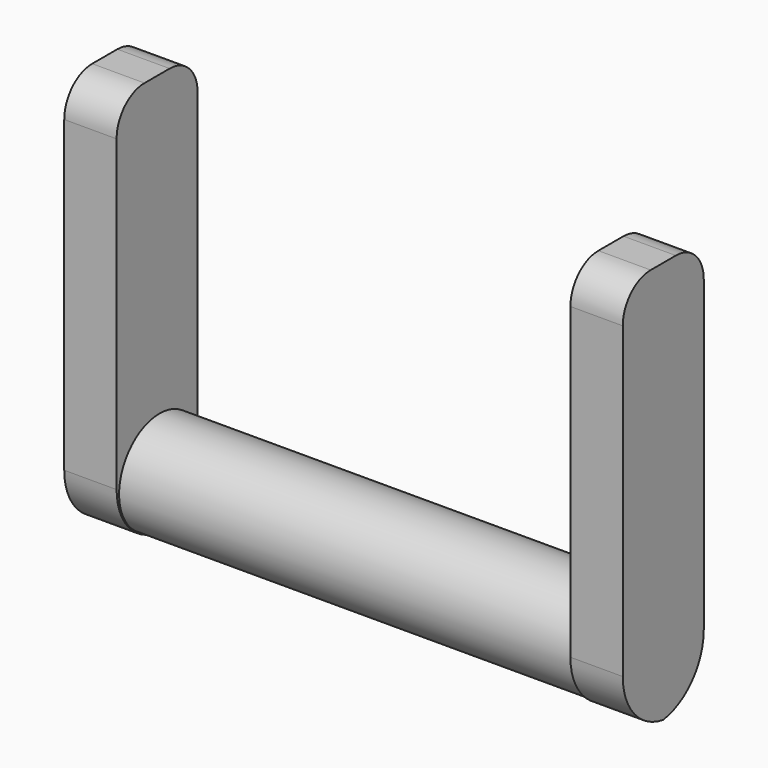
from build123d import *

# Parameters (mm, degrees)
F0_R          = 1.8415
F1_DEPTH      = 16.51
F2_W          = 1.905
F2_H          = 3.683
F3_DEPTH      = 12.7
F3_DEPTH_BACK = 1.96215
F4_T1_DEPTH   = 12.7
F4_T3_DEPTH   = 7.3025
F4_T5_DEPTH   = 12.7
F4_T7_DEPTH   = 7.3025
F5_R          = 1.27


# Not quite as in the source:
# - a fillet or chamfer that OpenCascade refuses, or shapes differently, is made with other operations: its cross-section is extruded or revolved along the edge and cut away or added


with BuildPart() as f1:
    # F0 (on Right) → F1 (new body)
    with BuildSketch(Plane.YZ):
        Circle(F0_R)
    extrude(amount=F1_DEPTH)

    # F2 (on Top) → F3 (join, two sides)
    with BuildSketch(Plane.XY) as f3_sk:
        with Locations((17.4625, -0.1134487624)):
            Rectangle(F2_W, F2_H)
        with Locations((-0.9525, -0.1134487624)):
            Rectangle(F2_W, F2_H)
    extrude(amount=F3_DEPTH)
    extrude(f3_sk.sketch, amount=-F3_DEPTH_BACK)

    # F4: fillet of radius 2.159 on 4 edges, made by hand

    # F4_s2 → F4_t1 (cut)
    with BuildSketch(Plane.YZ.offset(11.1125)):
        with BuildLine():
            ThreePointArc((0.2040512376, -1.96215), (-1.322592303, -1.3297935406), (-1.9549487624, 0.19685))
            Line((-1.9549487624, 0.19685), (-1.9549487624, -1.96215))
            Line((-1.9549487624, -1.96215), (0.2040512376, -1.96215))
        make_face()
    extrude(amount=F4_T1_DEPTH, mode=Mode.SUBTRACT)

    # F4_s4 → F4_t3 (cut)
    with BuildSketch(Plane.YZ.offset(16.51)):
        with BuildLine():
            ThreePointArc((1.7280512376, 0.19685), (1.0956947782, -1.3297935406), (-0.4309487624, -1.96215))
            Line((-0.4309487624, -1.96215), (1.7280512376, -1.96215))
            Line((1.7280512376, -1.96215), (1.7280512376, 0.19685))
        make_face()
    extrude(amount=F4_T3_DEPTH, mode=Mode.SUBTRACT)

    # F4_s6 → F4_t5 (cut)
    with BuildSketch(Plane.YZ.offset(-7.3025)):
        with BuildLine():
            ThreePointArc((-1.9549487624, 0.19685), (-1.322592303, -1.3297935406), (0.2040512376, -1.96215))
            Line((0.2040512376, -1.96215), (-1.9549487624, -1.96215))
            Line((-1.9549487624, -1.96215), (-1.9549487624, 0.19685))
        make_face()
    extrude(amount=F4_T5_DEPTH, mode=Mode.SUBTRACT)

    # F4_s8 → F4_t7 (cut)
    with BuildSketch(Plane.YZ.offset(-7.3025)):
        with BuildLine():
            ThreePointArc((1.7280512376, 0.19685), (1.0956947782, -1.3297935406), (-0.4309487624, -1.96215))
            Line((-0.4309487624, -1.96215), (1.7280512376, -1.96215))
            Line((1.7280512376, -1.96215), (1.7280512376, 0.19685))
        make_face()
    extrude(amount=F4_T7_DEPTH, mode=Mode.SUBTRACT)

    # F5
    f5_edges = [f1.edges().sort_by_distance(p)[0] for p in [
        (-0.9525, -1.954949, 12.7),
        (-0.9525, 1.728051, 12.7),
        (17.4625, 1.728051, 12.7),
        (17.4625, -1.954949, 12.7),
    ]]
    fillet(f5_edges, radius=F5_R)


solid = f1.part
